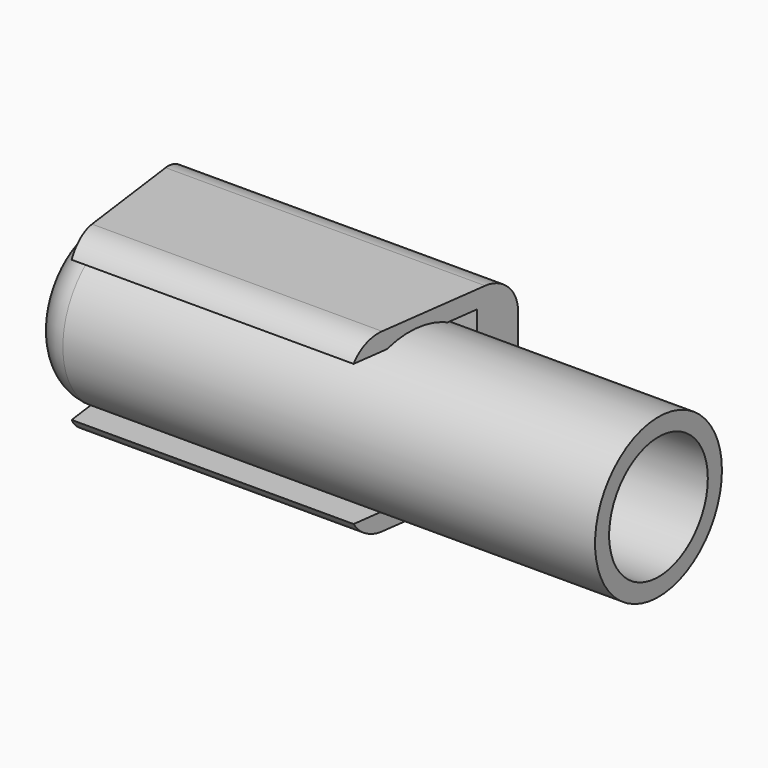
from build123d import *

# Parameters (mm, degrees)
F0_W        = 50.8
F0_H        = 25.4
F1_DEPTH    = 25.4
F2_T        = -2.54
F3_T1_DEPTH = 223.4557170743
F4_T1_DEPTH = 72.8133333333
F4_T3_DEPTH = 62.6370452561
F5_R        = 11.43
F6_DEPTH    = 81.788
F7_R        = 5.08
F8_T        = -2.54


# Not quite as in the source:
# - a fillet or chamfer that OpenCascade refuses, or shapes differently, is made with other operations: its cross-section is extruded or revolved along the edge and cut away or added


with BuildPart() as f1:
    # F0 (on Front) → F1 (new body)
    with BuildSketch(Plane.XZ):
        with Locations((25.4, 12.7)):
            Rectangle(F0_W, F0_H)
    extrude(amount=F1_DEPTH)

    # F2
    f2_openings = [f1.faces().sort_by_distance(p)[0] for p in [
        (25.4, -25.4, 12.7),
    ]]
    offset(amount=F2_T, openings=f2_openings)

    # F3: chamfer of 5.08 x 38.1 on 2 edges, made by hand

    # F3_s2 → F3_t1 (cut)
    with BuildSketch(Plane.XY.offset(-99.0278585372)):
        Polygon((50.8, 12.7), (45.72, -25.4), (50.8, -25.4), align=None)
        Polygon((0, 12.7), (5.08, -25.4), (0, -25.4), align=None)
    extrude(amount=F3_T1_DEPTH, mode=Mode.SUBTRACT)

    # F4: fillet of radius 5.08 on 4 edges, made by hand

    # F4_s2 → F4_t1 (cut)
    with BuildSketch(Plane.YZ.offset(-11.0066666667)):
        with BuildLine():
            ThreePointArc((-5.08, 25.4), (-1.4878975516, 23.9121024484), (0, 20.32))
            Line((0, 20.32), (0, 25.4))
            Line((0, 25.4), (-5.08, 25.4))
        make_face()
        with BuildLine():
            ThreePointArc((0, 5.08), (-1.4878975516, 1.4878975516), (-5.08, 0))
            Line((-5.08, 0), (0, 0))
            Line((0, 0), (0, 5.08))
        make_face()
    extrude(amount=F4_T1_DEPTH, mode=Mode.SUBTRACT)

    # F4_s4 → F4_t3 (cut)
    with BuildSketch(Plane.YZ.offset(-5.9185226281)):
        with BuildLine():
            ThreePointArc((-21.0005909488, 0), (-23.5405909488, 0.6805909488), (-25.4, 2.54))
            Line((-25.4, 2.54), (-25.4, 0))
            Line((-25.4, 0), (-21.0005909488, 0))
        make_face()
        with BuildLine():
            ThreePointArc((-21.0005909488, 25.4), (-23.5405909488, 24.7194090512), (-25.4, 22.86))
            Line((-25.4, 22.86), (-25.4, 25.4))
            Line((-25.4, 25.4), (-21.0005909488, 25.4))
        make_face()
    extrude(amount=F4_T3_DEPTH, mode=Mode.SUBTRACT)


with BuildPart() as f6:
    # F5 (on Right) → F6 (new body)
    with BuildSketch(Plane.YZ):
        with Locations((-15.5496466905, 12.4397175387)):
            Circle(F5_R)
    extrude(amount=F6_DEPTH)

    # F7
    f7_edges = [f6.edges().sort_by_distance(p)[0] for p in [
        (0, -26.979647, 12.439718),
    ]]
    fillet(f7_edges, radius=F7_R)

    # F8
    f8_openings = [f6.faces().sort_by_distance(p)[0] for p in [
        (81.788, -15.549647, 12.439718),
    ]]
    offset(amount=F8_T, openings=f8_openings)


solid = Compound([f1.part, f6.part])
